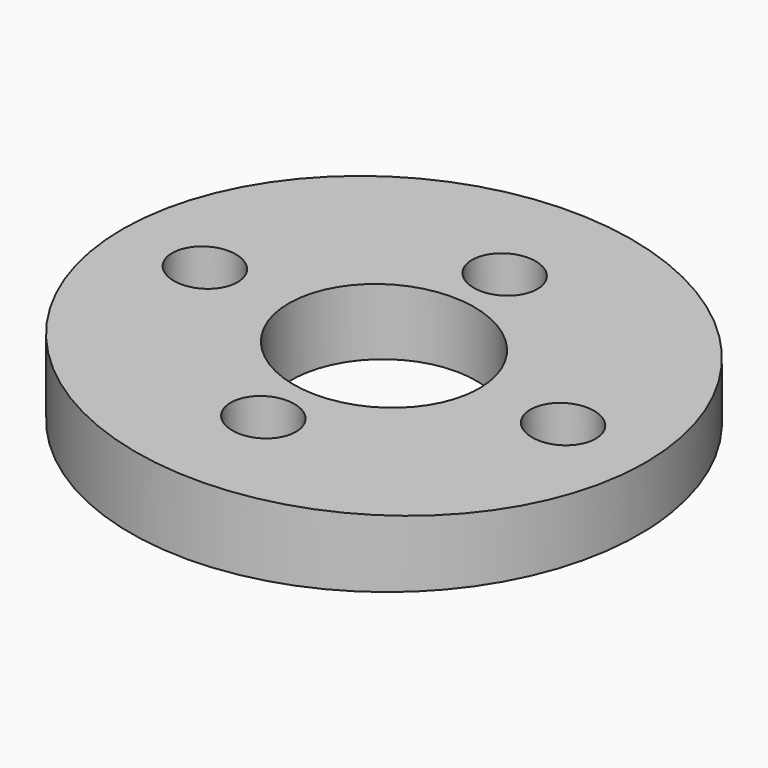
from build123d import *

# Parameters (mm, degrees)
F0_R     = 14
F0_R_2   = 1.75
F0_R_3   = 5.1
F1_DEPTH = 10
F6_DEPTH = 40


with BuildPart() as f1:
    # F0 (on Top) → F1 (new body)
    with BuildSketch(Plane.XY):
        Circle(F0_R)
        with Locations((0, -8)):
            Circle(F0_R_2, mode=Mode.SUBTRACT)
        with Locations((-9.5, 0)):
            Circle(F0_R_2, mode=Mode.SUBTRACT)
        Circle(F0_R_3, mode=Mode.SUBTRACT)
        with Locations((9.5, 0)):
            Circle(F0_R_2, mode=Mode.SUBTRACT)
        with Locations((0, 8)):
            Circle(F0_R_2, mode=Mode.SUBTRACT)
    extrude(amount=F1_DEPTH)

    # F5 (on face) → F6 (intersect)
    with BuildSketch(Plane(origin=(17.6564226245, -17.6564226245, -1.2253490154), x_dir=(0.7045622489, 0.7079556371, -0.0488963521), z_dir=(0.706256905, -0.706256905, -0.0490139606))):
        Polygon((-42.6054166353, 4.1487906781), (-42.3605061004, -0.8479598781), (14.9219552549, 1.9596804268), (14.7750896798, 4.9560833541), align=None)
        Polygon((14.7750896798, 4.9560833541), (14.9219552549, 1.9596804268), (100.7277084193, 6.1653602332), align=None)
    extrude(amount=-F6_DEPTH, mode=Mode.INTERSECT)


solid = f1.part
